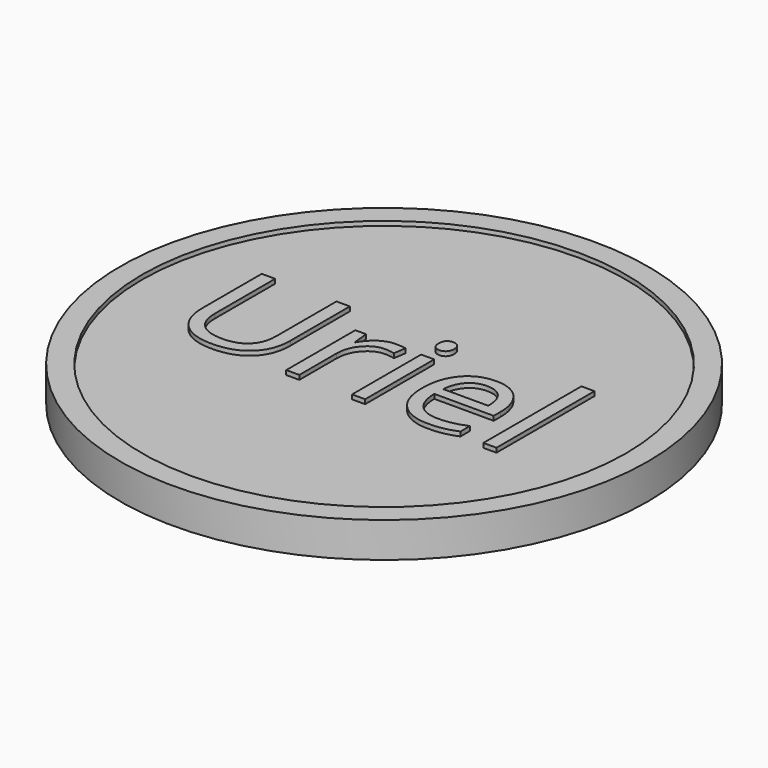
from build123d import *

# Parameters (mm, degrees)
F0_R         = 38.1
F1_DEPTH     = 3.81
F2_R         = 38.1
F2_R_2       = 34.925
F2_W         = 5.08
F2_H         = 5.08
F3_DEPTH     = 0.635
F4_TEXT_SIZE = 23.2793928111
F5_DEPTH     = 0.635
F6_R         = 38.1
F6_R_2       = 34.925
F7_DEPTH     = 0.635


# Not quite as in the source:
# - Text() gives the source's letters only with a copy of the font that has no kerning and outlines rounded to 1/6400 em; it was checked with that copy


with BuildPart() as f1:
    # F0 (on Top) → F1 (new body)
    with BuildSketch(Plane.XY):
        Circle(F0_R)
    extrude(amount=F1_DEPTH)

    # F2 (on Top) → F3 (join)
    with BuildSketch(Plane.XY):
        Circle(F2_R)
        Circle(F2_R_2, mode=Mode.SUBTRACT)
        Polygon((-13.97, 3.81), (-13.97, 8.89), (-20.32, 8.89), (-25.4, 3.81), (-25.4, -11.43), (-20.32, -16.51), (-5.08, -16.51), (0, -11.43), (0, -7.62), (-5.08, -7.62), (-5.08, -11.43), (-20.32, -11.43), (-20.32, 3.81), align=None)
        Polygon((-13.97, 8.89), (-8.89, 8.89), (-8.89, 14.1049223021), (3.7975644068, 14.1049223021), (3.7975644068, -7.62), (11.1271005431, -7.62), (11.1271005431, -2.54), (8.5871005431, -2.54), (8.8775644068, 13.2586937398), (3.7975644068, 18.3386937398), (-8.89, 18.3386937398), (-13.97, 13.2586937398), align=None)
        Polygon((-8.89, -7.62), (-8.89, 3.81), (-13.97, 3.81), (-13.97, -2.54), (-16.51, -2.54), (-16.51, -7.62), align=None)
        Polygon((0, 0), (0, 3.81), (-5.08, 8.89), (-8.89, 8.89), (-8.89, 3.81), (-5.08, 3.81), (-5.08, 0), align=None)
        with Locations((-11.43, 6.35)):
            Rectangle(F2_W, F2_H)
    extrude(amount=-F3_DEPTH)

    # F4 (on face) → F5 (join)
    with BuildSketch(Plane.XY.offset(3.81)):
        with Locations((-26.6281504629, -8.0533134456)):
            Text('Uriel', F4_TEXT_SIZE, font='Open Sans', text_align=(TextAlign.LEFT, TextAlign.BOTTOM))
    extrude(amount=F5_DEPTH)

    # F6 (on face) → F7 (join)
    with BuildSketch(Plane.XY.offset(3.81)):
        Circle(F6_R)
        Circle(F6_R_2, mode=Mode.SUBTRACT)
    extrude(amount=F7_DEPTH)


solid = f1.part
